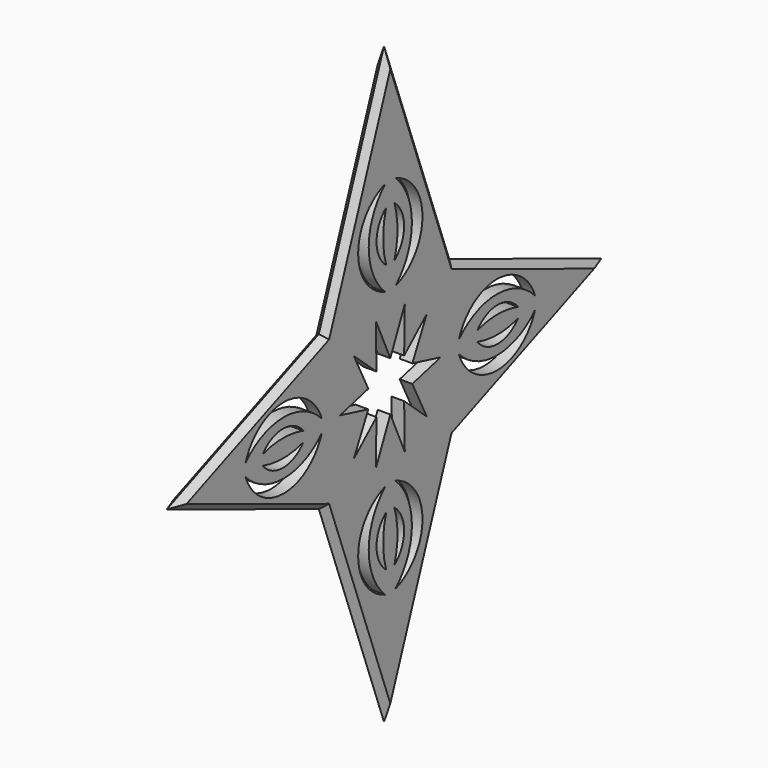
from build123d import *

# Parameters (mm, degrees)
F1_DEPTH = 3
F2_SIZE  = 1.49999
F4_DEPTH = 25
F6_DEPTH = 3.001
F8_COUNT = 4


# Not quite as in the source:
# - a fillet or chamfer is up to 0.001 mm smaller than in the source, because OpenCascade refuses the exact size


with BuildPart() as f1:
    # F0 (on Right) → F1 (new body)
    with BuildSketch(Plane.YZ):
        Polygon((-19.3618498743, -18.3178298175), (0, -70.7087218761), (19.3618498743, -18.3178298175), (64.5395070314, 0), (19.3618498743, 18.3178298175), (0, 70.7087218761), (-19.3618498743, 18.3178298175), (-64.5395070314, 0), align=None)
    extrude(amount=F1_DEPTH)

    # F2 (size 1.5 in the source; OpenCascade refuses exactly that, so slightly less here)
    f2_edges = [f1.edges().sort_by_distance(p)[0] for p in [
        (3, -41.950678, 9.158915),
        (3, -9.680925, 44.513276),
        (0, -9.680925, 44.513276),
        (0, -41.950678, 9.158915),
        (0, -41.950678, -9.158915),
        (3, -41.950678, -9.158915),
        (0, -9.680925, -44.513276),
        (3, -9.680925, -44.513276),
        (3, 9.680925, -44.513276),
        (0, 9.680925, -44.513276),
        (3, 41.950678, -9.158915),
        (0, 41.950678, -9.158915),
        (0, 9.680925, 44.513276),
        (3, 9.680925, 44.513276),
        (3, 41.950678, 9.158915),
        (0, 41.950678, 9.158915),
    ]]
    chamfer(f2_edges, length=F2_SIZE)

    # F3 (on Right) → F4 (cut)
    with BuildSketch(Plane.YZ):
        Polygon((-4.2971530929, -15.4137015343), (0, -5.8852313086), (4.2971530929, -15.4137015343), (4.1103190742, -4.7642351128), (10.8362995088, -10.7428822666), (6.5391454846, -2.1485765465), (14.94661998, 0), (6.5391454846, 2.1485765465), (10.8362995088, 10.7428822666), (4.1103190742, 4.7642351128), (4.2971530929, 15.4137015343), (0, 5.8852313086), (-4.2971530929, 15.4137015343), (-4.1103190742, 4.7642351128), (-10.8362995088, 10.7428822666), (-6.5391454846, 2.1485765465), (-14.94661998, 0), (-6.5391454846, -2.1485765465), (-10.8362995088, -10.7428822666), (-4.1103190742, -4.7642351128), align=None)
    extrude(amount=F4_DEPTH, mode=Mode.SUBTRACT)

    # F5 (on Right) → F6 (cut, through all)
    with BuildSketch(Plane.YZ):
        with BuildLine():
            ThreePointArc((-1.5215650201, -20.3531272709), (-9.5569240867, -31.6740609705), (-1.5215650201, -42.9949946702))
            ThreePointArc((-1.5215650201, -42.9949946702), (-6.4116749119, -31.6740609705), (-1.5215650201, -20.3531272709))
        make_face()
        with BuildLine():
            ThreePointArc((-1.2058431748, -25.8382316679), (-4.0993778142, -31.8839969113), (-1.2058431748, -37.9297621548))
            ThreePointArc((-1.2058431748, -37.9297621548), (-2.1323484034, -31.8839969113), (-1.2058431748, -25.8382316679))
        make_face()
        with BuildLine():
            ThreePointArc((1.5215650201, -20.3531272709), (6.4116749119, -31.6740609705), (1.5215650201, -42.9949946702))
            ThreePointArc((1.5215650201, -42.9949946702), (9.5569240867, -31.6740609705), (1.5215650201, -20.3531272709))
        make_face()
        with BuildLine():
            ThreePointArc((1.2058431748, -25.8382316679), (2.1323484034, -31.8839969113), (1.2058431748, -37.9297621548))
            ThreePointArc((1.2058431748, -37.9297621548), (4.0993778142, -31.8839969113), (1.2058431748, -25.8382316679))
        make_face()
    f6 = extrude(amount=F6_DEPTH, mode=Mode.SUBTRACT)

    # F8: F6 ×4 about axis
    f8_axis = Axis((-24.6906243265, 0, 0), (-1, 0, 0))
    for i in range(1, F8_COUNT):
        add(f6.rotate(f8_axis, i * 360 / F8_COUNT), mode=Mode.SUBTRACT)


solid = f1.part
